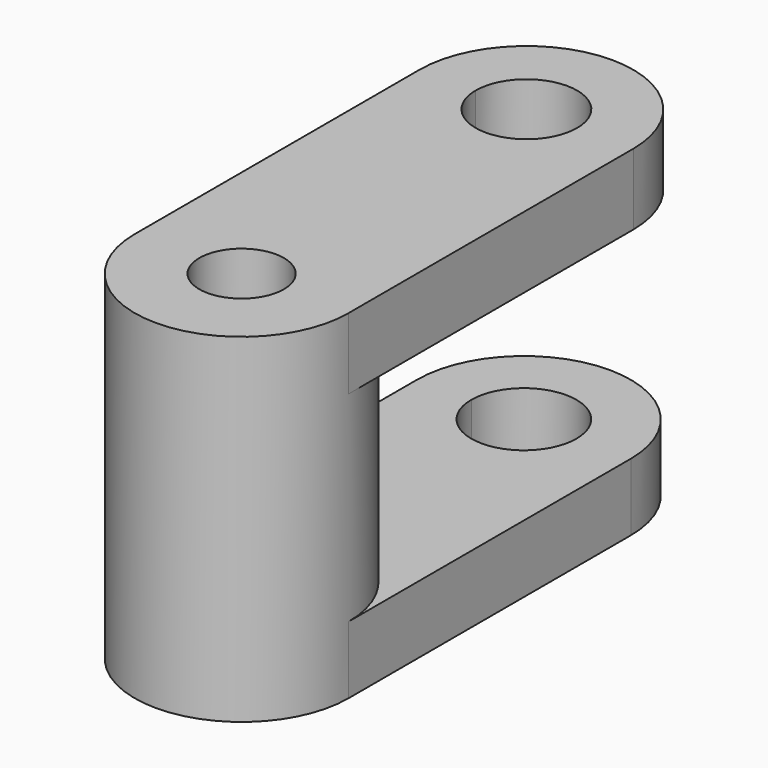
from build123d import *

# Parameters (mm, degrees)
F0_R     = 28.9961675247
F0_R_2   = 11.4701678976
F1_DEPTH = 45.974
F3_DEPTH = 19.304
F5_DEPTH = 18.288


# Not quite as in the source:
# - ends of sketch curves that miss each other by under 0.0002 mm in the source are joined


with BuildPart() as f1:
    # F0 (on Top) → F1 (new body, symmetric)
    with BuildSketch(Plane.XY):
        Circle(F0_R)
        Circle(F0_R_2, mode=Mode.SUBTRACT)
    extrude(amount=F1_DEPTH, both=True)

    # F2 (on face) → F3 (join)
    with BuildSketch(Plane.XY.offset(45.974)):
        with BuildLine():
            ThreePointArc((-28.9961675247, 96.5353175998), (0, 67.5391500751), (28.9961675247, 96.5353175998))
            ThreePointArc((28.9961675247, 96.5353175998), (0, 125.5314851244), (-28.9961675247, 96.5353175998))
        make_face()
        with BuildLine():
            ThreePointArc((-13.7561708689, 96.5353175998), (0, 110.2914884686), (13.7561708689, 96.5353175998))
            ThreePointArc((13.7561708689, 96.5353175998), (0, 82.7791500751), (-13.7561708689, 96.5353175998))
        make_face(mode=Mode.SUBTRACT)
        with BuildLine():
            Line((-28.9961675247, 96.5353175998), (-28.9961675247, 0))
            ThreePointArc((-28.9961675247, 0), (0, 28.9961675247), (28.9961675247, 0))
            Line((28.9961675247, 0), (28.9961675247, 96.5353175998))
            ThreePointArc((28.9961675247, 96.5353175998), (0, 67.5391500751), (-28.9961675247, 96.5353175998))
        make_face()
    extrude(amount=-F3_DEPTH)

    # F4 (on face) → F5 (join)
    with BuildSketch(Plane(origin=(0, 0, -45.974), x_dir=(1, 0, 0), z_dir=(0, 0, -1))):
        with BuildLine():
            Line((28.9961675247, -95.6837162375), (28.9961675247, 0))
            ThreePointArc((28.9961675247, 0), (0, -28.9961675247), (-28.9961675247, 0))
            Line((-28.9961675247, 0), (-28.9961675247, -95.6837162375))
            ThreePointArc((-28.9961675247, -95.6837162375), (0, -66.6875487129), (28.9961675247, -95.6837162375))
        make_face()
        with BuildLine():
            ThreePointArc((-28.9961675247, -95.6837162375), (0, -124.6798837622), (28.9961675247, -95.6837162375))
            ThreePointArc((28.9961675247, -95.6837162375), (0, -66.6875487129), (-28.9961675247, -95.6837162375))
        make_face()
        with BuildLine():
            ThreePointArc((14.2641663551, -95.6837162375), (0, -109.9478825927), (-14.2641663551, -95.6837162375))
            ThreePointArc((-14.2641663551, -95.6837162375), (0, -81.4195498824), (14.2641663551, -95.6837162375))
        make_face(mode=Mode.SUBTRACT)
    extrude(amount=-F5_DEPTH)


solid = f1.part
